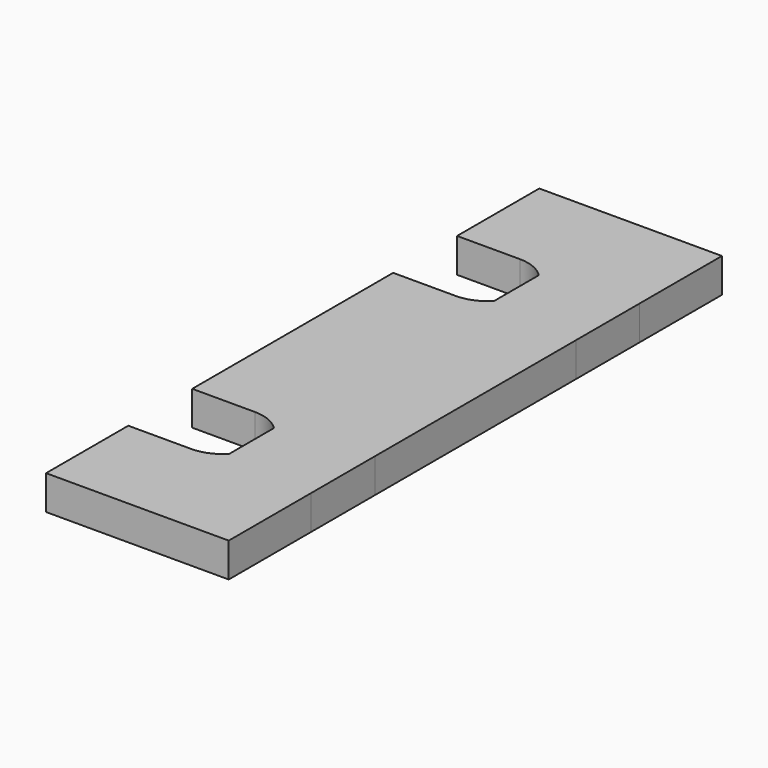
from build123d import *

# Parameters (mm, degrees)
F1_DEPTH = 1.5


# Not quite as in the source:
# - ends of sketch curves that miss each other by under 0.0002 mm in the source are joined


with BuildPart() as f1:
    # F0 (on Top) → F1 (new body)
    with BuildSketch(Plane.XY):
        Polygon((-34.6231374532, -30.5467036664), (-34.6231374532, -35.0467036664), (-31.8731374532, -35.0467036664), (-30.6230945961, -35.0467036664), (-26.6231374532, -35.0467036664), (-26.6231374532, -30.5467036664), (-30.6230517389, -30.5467036664), align=None)
        with BuildLine():
            Line((-30.6230945961, -35.0467036664), (-31.8731374532, -35.0467036664))
            ThreePointArc((-31.8731374532, -35.0467036664), (-31.1952175422, -35.1833094776), (-30.6231474562, -35.5718611088))
            Line((-30.6231474562, -35.5718611088), (-30.6230945961, -35.0467036664))
        make_face()
        with BuildLine():
            Line((-26.6231374532, -35.0467036664), (-30.6230945961, -35.0467036664))
            Line((-30.6230945961, -35.0467036664), (-30.6231474562, -35.5718611088))
            ThreePointArc((-30.6231474562, -35.5718611088), (-30.1230517371, -36.796737), (-30.6231941178, -38.0215938389))
            Line((-30.6231941178, -38.0215938389), (-30.6232041199, -38.5467036666))
            Line((-30.6232041199, -38.5467036666), (-26.6232041199, -38.5467036666))
            Line((-26.6232041199, -38.5467036666), (-26.6231374532, -35.0467036664))
        make_face()
        with BuildLine():
            ThreePointArc((-30.6231941178, -38.0215938389), (-30.1230517371, -36.796737), (-30.6231474562, -35.5718611088))
            Line((-30.6231474562, -35.5718611088), (-30.6231941178, -38.0215938389))
        make_face()
        with BuildLine():
            Line((-30.6232041199, -38.5467036666), (-30.6231941178, -38.0215938389))
            ThreePointArc((-30.6231941178, -38.0215938389), (-31.1951692504, -38.410077566), (-31.8729660246, -38.5467036666))
            Line((-31.8729660246, -38.5467036666), (-30.6232041199, -38.5467036666))
        make_face()
        Polygon((-26.6234136437, -49.5467036666), (-26.6232041199, -38.5467036666), (-30.6232041199, -38.5467036666), (-30.6234136437, -49.5467036665), align=None)
        Polygon((-30.6234136437, -49.5467036665), (-30.6232041199, -38.5467036666), (-31.8729660246, -38.5467036666), (-34.6229279294, -38.5467036666), (-34.6231374532, -49.5467036664), (-31.8734136439, -49.5467036665), align=None)
        with BuildLine():
            Line((-26.6234803104, -53.0467036664), (-26.6234136437, -49.5467036666))
            Line((-26.6234136437, -49.5467036666), (-30.6234136437, -49.5467036665))
            Line((-30.6234136437, -49.5467036665), (-30.623423649, -50.0719826043))
            ThreePointArc((-30.623423649, -50.0719826043), (-30.1234469771, -51.2967369998), (-30.6234703059, -52.5214723478))
            Line((-30.6234703059, -52.5214723478), (-30.6234803104, -53.0467036664))
            Line((-30.6234803104, -53.0467036664), (-26.6234803104, -53.0467036664))
        make_face()
        with BuildLine():
            Line((-30.623423649, -50.0719826043), (-30.6234136437, -49.5467036665))
            Line((-30.6234136437, -49.5467036665), (-31.8734136439, -49.5467036665))
            ThreePointArc((-31.8734136439, -49.5467036665), (-31.1954794965, -49.6833654824), (-30.623423649, -50.0719826043))
        make_face()
        Polygon((-26.6235660246, -57.5467036664), (-26.6234803104, -53.0467036664), (-30.6234803104, -53.0467036664), (-31.8734803104, -53.0467036664), (-34.6234803104, -53.0467036664), (-34.6234803104, -57.5467036664), align=None)
        with BuildLine():
            ThreePointArc((-30.6234703059, -52.5214723478), (-30.1234469771, -51.2967369998), (-30.623423649, -50.0719826043))
            Line((-30.623423649, -50.0719826043), (-30.6234703059, -52.5214723478))
        make_face()
        with BuildLine():
            Line((-31.8734803104, -53.0467036664), (-30.6234803104, -53.0467036664))
            Line((-30.6234803104, -53.0467036664), (-30.6234703059, -52.5214723478))
            ThreePointArc((-30.6234703059, -52.5214723478), (-31.1955409574, -52.9100676767), (-31.8734803104, -53.0467036665))
        make_face()
    extrude(amount=F1_DEPTH)


solid = f1.part
